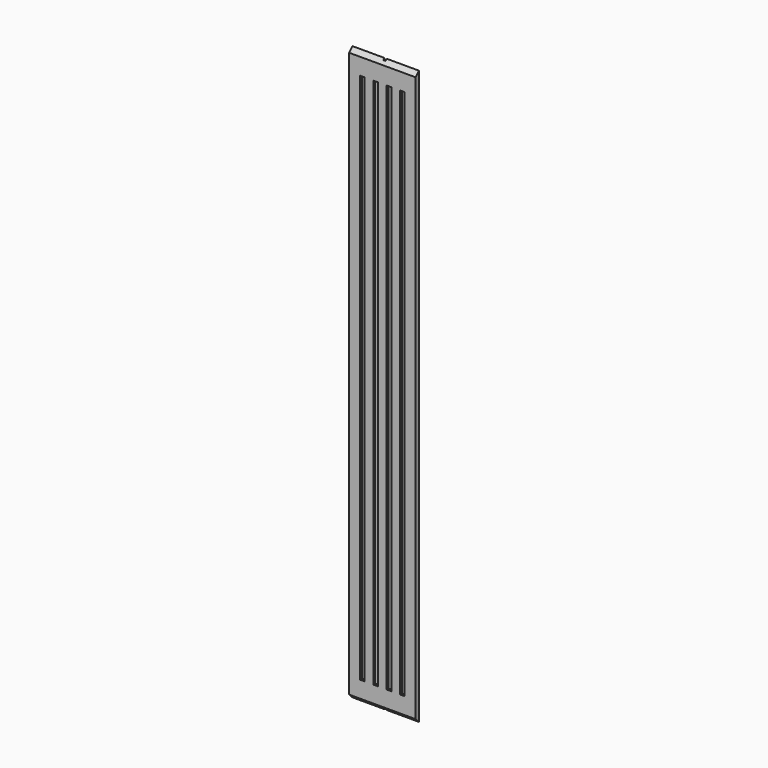
from build123d import *

# Parameters (mm, degrees)
F0_W     = 304.8
F0_H     = 2628.9
F1_DEPTH = 19.05
F2_SIZE  = 19.04999
F3_W     = 21.082
F3_H     = 2438.4
F4_DEPTH = 10.16
F5_W     = 9.525
F5_H     = 95.25
F6_DEPTH = 6.35


# Not quite as in the source:
# - a fillet or chamfer is up to 0.001 mm smaller than in the source, because OpenCascade refuses the exact size


with BuildPart() as f1:
    # F0 (on Front) → F1 (new body)
    with BuildSketch(Plane.XZ):
        with Locations((-2.8532538563, 1186.9243339048)):
            Rectangle(F0_W, F0_H)
    extrude(amount=F1_DEPTH)

    # F2 (size 19.05 in the source; OpenCascade refuses exactly that, so slightly less here)
    f2_edges = [f1.edges().sort_by_distance(p)[0] for p in [
        (-2.853254, -19.05, 2501.374334),
        (-2.853254, -19.05, -127.525666),
    ]]
    chamfer(f2_edges, length=F2_SIZE)

    # F3 (on face) → F4 (cut)
    with BuildSketch(Plane.XZ.offset(19.05)):
        with Locations((-94.2932538563, 1186.9243339048)):
            Rectangle(F3_W, F3_H)
        with Locations((-33.3332538563, 1186.9243339048)):
            Rectangle(F3_W, F3_H)
        with Locations((27.6267461437, 1186.9243339048)):
            Rectangle(F3_W, F3_H)
        with Locations((88.5867461437, 1186.9243339048)):
            Rectangle(F3_W, F3_H)
    extrude(amount=-F4_DEPTH, mode=Mode.SUBTRACT)

    # F5 (on face) → F6 (cut)
    with BuildSketch(Plane(origin=(0, 0, 0), x_dir=(-1, 0, 0), z_dir=(0, 1, 0))):
        Polygon((-1.9092461437, 2406.1243339048), (-99.1277461437, 2406.1243339048), (-99.1277461437, 2396.5993339048), (104.8342538563, 2396.5993339048), (104.8342538563, 2406.1243339048), (7.6157538563, 2406.1243339048), align=None)
        with Locations((2.8532538563, 2453.7493339048)):
            Rectangle(F5_W, F5_H)
        with Locations((2.8532538563, -79.9006660952)):
            Rectangle(F5_W, F5_H)
        Polygon((-99.1277461437, -32.2756660952), (-1.9092461437, -32.2756660952), (7.6157538563, -32.2756660952), (104.8342538563, -32.2756660952), (104.8342538563, -22.7506660952), (-99.1277461437, -22.7506660952), align=None)
    extrude(amount=-F6_DEPTH, mode=Mode.SUBTRACT)


solid = f1.part
